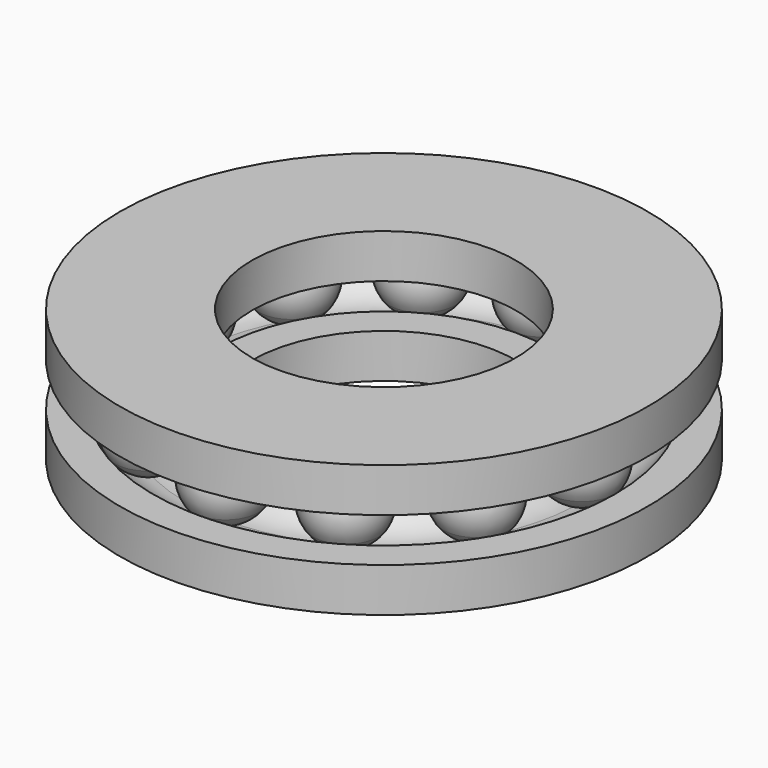
from build123d import *

# Parameters (mm, degrees)
F3_COUNT = 12


with BuildPart() as f1:
    # F0 (on Front) → F1 (revolve)
    with BuildSketch(Plane.XZ):
        with BuildLine():
            ThreePointArc((-17.4974131955, 6.6622055622), (-18, 5), (-17.4974131955, 3.3377944378))
            ThreePointArc((-17.4974131955, 3.3377944378), (-16.4165774447, 2.3555135956), (-15, 2))
            Line((-15, 2), (-15, 8))
            ThreePointArc((-15, 8), (-16.4165774447, 7.6444864044), (-17.4974131955, 6.6622055622))
        make_face()
    revolve(axis=Axis((-15, 0, 5), (0, 0, -1)))


with BuildPart() as f2:
    # F0 (on Front) → F2 (revolve)
    with BuildSketch(Plane.XZ):
        with BuildLine():
            Line((-20, 6.6622055622), (-17.4974131955, 6.6622055622))
            ThreePointArc((-17.4974131955, 6.6622055622), (-16.4165774447, 7.6444864044), (-15, 8))
            ThreePointArc((-15, 8), (-13.5834225553, 7.6444864044), (-12.5025868045, 6.6622055622))
            Line((-12.5025868045, 6.6622055622), (-10, 6.6622055622))
            Line((-10, 6.6622055622), (-10, 10))
            Line((-10, 10), (-20, 10))
            Line((-20, 10), (-20, 6.6622055622))
        make_face()
    revolve(axis=Axis((0, 0, -8.1000216305), (0, 0, -1)))


with BuildPart() as f2b:
    # F0 (on Front) → F2, piece 2 (revolve)
    with BuildSketch(Plane.XZ):
        with BuildLine():
            Line((-20, 0), (-10, 0))
            Line((-10, 0), (-10, 3.3377944378))
            Line((-10, 3.3377944378), (-12.5025868045, 3.3377944378))
            ThreePointArc((-12.5025868045, 3.3377944378), (-13.5834225553, 2.3555135956), (-15, 2))
            ThreePointArc((-15, 2), (-16.4165774447, 2.3555135956), (-17.4974131955, 3.3377944378))
            Line((-17.4974131955, 3.3377944378), (-20, 3.3377944378))
            Line((-20, 3.3377944378), (-20, 0))
        make_face()
    revolve(axis=Axis((0, 0, -8.1000216305), (0, 0, -1)))


with BuildPart() as f3_1:
    # F3: instance of F1
    add(f1.part.rotate(Axis((0, 0, -8.1000216305), (0, 0, -1)), 1 * 360 / F3_COUNT))


with BuildPart() as f3_2:
    # F3: instance of F1
    add(f1.part.rotate(Axis((0, 0, -8.1000216305), (0, 0, -1)), 2 * 360 / F3_COUNT))


with BuildPart() as f3_3:
    # F3: instance of F1
    add(f1.part.rotate(Axis((0, 0, -8.1000216305), (0, 0, -1)), 3 * 360 / F3_COUNT))


with BuildPart() as f3_4:
    # F3: instance of F1
    add(f1.part.rotate(Axis((0, 0, -8.1000216305), (0, 0, -1)), 4 * 360 / F3_COUNT))


with BuildPart() as f3_5:
    # F3: instance of F1
    add(f1.part.rotate(Axis((0, 0, -8.1000216305), (0, 0, -1)), 5 * 360 / F3_COUNT))


with BuildPart() as f3_6:
    # F3: instance of F1
    add(f1.part.rotate(Axis((0, 0, -8.1000216305), (0, 0, -1)), 6 * 360 / F3_COUNT))


with BuildPart() as f3_7:
    # F3: instance of F1
    add(f1.part.rotate(Axis((0, 0, -8.1000216305), (0, 0, -1)), 7 * 360 / F3_COUNT))


with BuildPart() as f3_8:
    # F3: instance of F1
    add(f1.part.rotate(Axis((0, 0, -8.1000216305), (0, 0, -1)), 8 * 360 / F3_COUNT))


with BuildPart() as f3_9:
    # F3: instance of F1
    add(f1.part.rotate(Axis((0, 0, -8.1000216305), (0, 0, -1)), 9 * 360 / F3_COUNT))


with BuildPart() as f3_10:
    # F3: instance of F1
    add(f1.part.rotate(Axis((0, 0, -8.1000216305), (0, 0, -1)), 10 * 360 / F3_COUNT))


with BuildPart() as f3_11:
    # F3: instance of F1
    add(f1.part.rotate(Axis((0, 0, -8.1000216305), (0, 0, -1)), 11 * 360 / F3_COUNT))


solid = Compound([f1.part, f2.part, f2b.part, f3_1.part, f3_2.part, f3_3.part, f3_4.part, f3_5.part, f3_6.part, f3_7.part, f3_8.part, f3_9.part, f3_10.part, f3_11.part])
